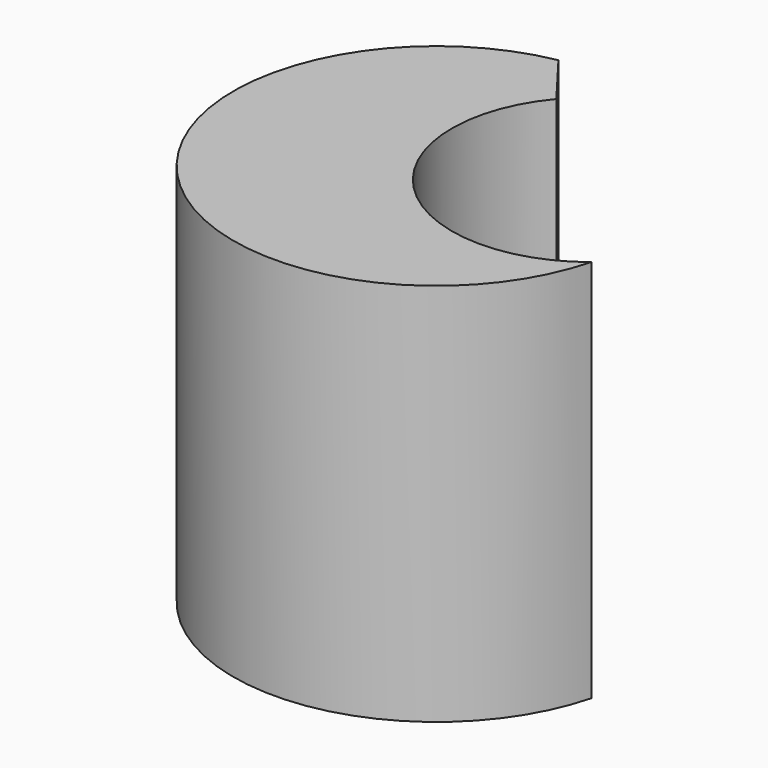
from build123d import *

# Parameters (mm, degrees)
F1_DEPTH = 36.576


with BuildPart() as f1:
    # F0 (on Top) → F1 (new body)
    with BuildSketch(Plane.XY):
        with BuildLine():
            ThreePointArc((11.8417274365, -10.3449132075), (-5.9441989082, -9.2653895435), (-6.6010553203, 8.5411566385))
            Line((-6.6010553203, 8.5411566385), (-10.3857247159, 13.5224955156))
            ThreePointArc((-10.3857247159, 13.5224955156), (-20.9717170118, -18.619915096), (11.8417274365, -10.3449132075))
        make_face()
    extrude(amount=F1_DEPTH)


solid = f1.part
